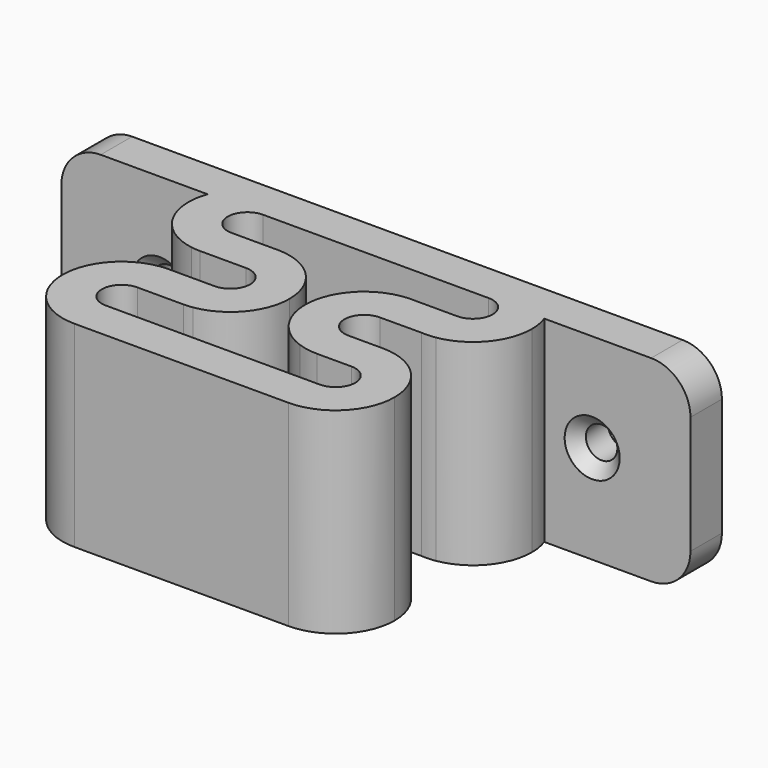
from build123d import *

# Parameters (mm, degrees)
F1_DEPTH       = 25
F2_W           = 5
F2_H           = 25
F3_DEPTH       = 40
F4_R           = 5
F6_D           = 4
F6_CSINK_D     = 7
F6_CSINK_ANGLE = 90


# Not quite as in the source:
# - a feature names something its author has since deleted; it is built from what else it names


with BuildPart() as f1:
    # F0 (on Top) → F1 (new body)
    with BuildSketch(Plane.XY):
        with BuildLine():
            ThreePointArc((-14.3421743065, 17.5), (-10.0120472875, 16.123724357), (-7.2711064946, 12.5))
            Line((-7.2711064946, 12.5), (7.2711064946, 12.5))
            ThreePointArc((7.2711064946, 12.5), (10.0120472875, 16.123724357), (14.3421743065, 17.5))
            Line((14.3421743065, 17.5), (-14.3421743065, 17.5))
        make_face()
        with BuildLine():
            ThreePointArc((-7.2711064946, -12.5), (-10.0120472875, -16.123724357), (-14.3421743065, -17.5))
            Line((-14.3421743065, -17.5), (12.8716113806, -17.5))
            ThreePointArc((12.8716113806, -17.5), (8.5414843617, -16.123724357), (5.8005435687, -12.5))
            Line((5.8005435687, -12.5), (-7.2711064946, -12.5))
        make_face()
        with BuildLine():
            ThreePointArc((14.3421743065, 17.5), (10.0120472875, 16.123724357), (7.2711064946, 12.5))
            Line((7.2711064946, 12.5), (14.3421743065, 12.5))
            ThreePointArc((14.3421743065, 12.5), (16.1099412594, 11.767766953), (16.8421743065, 10))
            ThreePointArc((16.8421743065, 10), (16.1099412594, 8.232233047), (14.3421743065, 7.5))
            Line((14.3421743065, 7.5), (8.5, 7.5))
            ThreePointArc((8.5, 7.5), (12.7884854356, 6.1529580422), (15.5364989199, 2.5957047116))
            ThreePointArc((15.5364989199, 2.5957047116), (20.052140795, 5.1372556412), (21.8421743065, 10))
            ThreePointArc((21.8421743065, 10), (19.6454751654, 15.3033008589), (14.3421743065, 17.5))
        make_face()
        with BuildLine():
            ThreePointArc((-14.3421743065, 7.5), (-16.8421743065, 10), (-14.3421743065, 12.5))
            Line((-14.3421743065, 12.5), (-7.2711064946, 12.5))
            ThreePointArc((-7.2711064946, 12.5), (-10.0120472875, 16.123724357), (-14.3421743065, 17.5))
            ThreePointArc((-14.3421743065, 17.5), (-21.8182098422, 10.5990765131), (-15.5364989199, 2.5957047116))
            ThreePointArc((-15.5364989199, 2.5957047116), (-12.7884854356, 6.1529580422), (-8.5, 7.5))
            Line((-8.5, 7.5), (-14.3421743065, 7.5))
        make_face()
        with BuildLine():
            ThreePointArc((-7.3056753865, 7.4042952884), (-7.9009234869, 7.4760355357), (-8.5, 7.5))
            ThreePointArc((-8.5, 7.5), (-12.7884854356, 6.1529580422), (-15.5364989199, 2.5957047116))
            ThreePointArc((-15.5364989199, 2.5957047116), (-14.9412508196, 2.5239644643), (-14.3421743065, 2.5))
            ThreePointArc((-14.3421743065, 2.5), (-10.0536888708, 3.8470419578), (-7.3056753865, 7.4042952884))
        make_face()
        with BuildLine():
            ThreePointArc((-1, 0), (-2.7900335114, 4.8627443588), (-7.3056753865, 7.4042952884))
            ThreePointArc((-7.3056753865, 7.4042952884), (-10.0536888708, 3.8470419578), (-14.3421743065, 2.5))
            Line((-14.3421743065, 2.5), (-8.5, 2.5))
            ThreePointArc((-8.5, 2.5), (-6.732233047, 1.767766953), (-6, 0))
            ThreePointArc((-6, 0), (-6.732233047, -1.767766953), (-8.5, -2.5))
            Line((-8.5, -2.5), (-14.3421743065, -2.5))
            ThreePointArc((-14.3421743065, -2.5), (-10.0536888708, -3.8470419578), (-7.3056753865, -7.4042952884))
            ThreePointArc((-7.3056753865, -7.4042952884), (-2.7900335114, -4.8627443588), (-1, 0))
        make_face()
        with BuildLine():
            ThreePointArc((-14.3421743065, -2.5), (-14.9412508196, -2.5239644643), (-15.5364989199, -2.5957047116))
            ThreePointArc((-15.5364989199, -2.5957047116), (-12.7884854356, -6.1529580422), (-8.5, -7.5))
            ThreePointArc((-8.5, -7.5), (-7.9009234869, -7.4760355357), (-7.3056753865, -7.4042952884))
            ThreePointArc((-7.3056753865, -7.4042952884), (-10.0536888708, -3.8470419578), (-14.3421743065, -2.5))
        make_face()
        with BuildLine():
            ThreePointArc((12.8716113806, -2.5), (8.7359797123, -3.7432795568), (5.9714803927, -7.0609198123))
            ThreePointArc((5.9714803927, -7.0609198123), (7.2168200812, -7.3894146789), (8.5, -7.5))
            ThreePointArc((8.5, -7.5), (12.6356316683, -6.2567204432), (15.4001309879, -2.9390801877))
            ThreePointArc((15.4001309879, -2.9390801877), (14.1547912994, -2.6105853211), (12.8716113806, -2.5))
        make_face()
        with BuildLine():
            ThreePointArc((8.5, 7.5), (7.9009234869, 7.4760355357), (7.3056753865, 7.4042952884))
            ThreePointArc((7.3056753865, 7.4042952884), (9.8321935715, 4.0074985381), (13.7956134511, 2.5199417628))
            ThreePointArc((13.7956134511, 2.5199417628), (14.6682639838, 2.5070923186), (15.5364989199, 2.5957047116))
            ThreePointArc((15.5364989199, 2.5957047116), (12.7884854356, 6.1529580422), (8.5, 7.5))
        make_face()
        with BuildLine():
            ThreePointArc((13.7956134511, 2.5199417628), (9.8321935715, 4.0074985381), (7.3056753865, 7.4042952884))
            ThreePointArc((7.3056753865, 7.4042952884), (1.0317000428, 0.6888365189), (5.9714803927, -7.0609198123))
            ThreePointArc((5.9714803927, -7.0609198123), (8.7359797123, -3.7432795568), (12.8716113806, -2.5))
            Line((12.8716113806, -2.5), (8.5, -2.5))
            ThreePointArc((8.5, -2.5), (6.0000044235, -0.0047029402), (8.4905941362, 2.4999823059))
            Line((8.4905941362, 2.4999823059), (13.7956134511, 2.5199417628))
        make_face()
        with BuildLine():
            ThreePointArc((-8.5, -7.5), (-12.7884854356, -6.1529580422), (-15.5364989199, -2.5957047116))
            ThreePointArc((-15.5364989199, -2.5957047116), (-21.8182098422, -10.5990765131), (-14.3421743065, -17.5))
            ThreePointArc((-14.3421743065, -17.5), (-10.0120472875, -16.123724357), (-7.2711064946, -12.5))
            Line((-7.2711064946, -12.5), (-14.3421743065, -12.5))
            ThreePointArc((-14.3421743065, -12.5), (-16.8421743065, -10), (-14.3421743065, -7.5))
            Line((-14.3421743065, -7.5), (-8.5, -7.5))
        make_face()
        with BuildLine():
            Line((12.8716113806, -12.5), (5.8005435687, -12.5))
            ThreePointArc((5.8005435687, -12.5), (8.5414843617, -16.123724357), (12.8716113806, -17.5))
            ThreePointArc((12.8716113806, -17.5), (18.1749122395, -15.3033008589), (20.3716113806, -10))
            ThreePointArc((20.3716113806, -10), (19.0040618311, -5.6822399936), (15.4001309879, -2.9390801877))
            ThreePointArc((15.4001309879, -2.9390801877), (12.6356316683, -6.2567204432), (8.5, -7.5))
            Line((8.5, -7.5), (12.8716113806, -7.5))
            ThreePointArc((12.8716113806, -7.5), (14.6393783336, -8.232233047), (15.3716113806, -10))
            ThreePointArc((15.3716113806, -10), (14.6393783336, -11.767766953), (12.8716113806, -12.5))
        make_face()
    extrude(amount=F1_DEPTH)

    # F2 (on Right) → F3 (join, symmetric)
    with BuildSketch(Plane.YZ):
        with Locations((15, 12.5)):
            Rectangle(F2_W, F2_H)
    extrude(amount=F3_DEPTH, both=True)

    # F4
    f4_edges = [f1.edges().sort_by_distance(p)[0] for p in [
        (40, 15, 0),
        (40, 15, 25),
        (-40, 15, 25),
        (-40, 15, 0),
    ]]
    fillet(f4_edges, radius=F4_R)

    # F6 (through all)
    with Locations(Plane.XZ.offset(-12.5)):
        with Locations((27.5, 12.5), (-27.5, 12.5)):
            CounterSinkHole(F6_D / 2, F6_CSINK_D / 2, counter_sink_angle=F6_CSINK_ANGLE)


solid = f1.part
